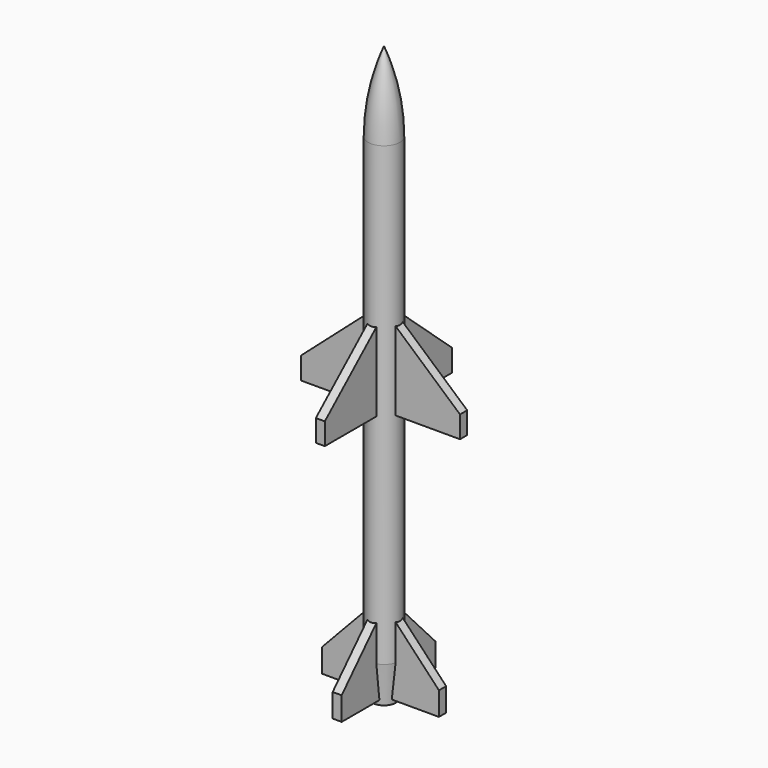
from build123d import *

# Parameters (mm, degrees)
F4_DEPTH     = 0.2
F5_COUNT     = 4
F7_DEPTH     = 17.9166666667
F8_T4_ANGLE  = 180
F8_S5_R      = 0.7048611111
F8_T6_DEPTH  = 2
F8_T10_DEPTH = 0.263819099
F8_S11_R     = 0.7048611111
F8_T12_DEPTH = 2
F8_T16_DEPTH = 0.263819099
F8_S17_R     = 0.7048611111
F8_T18_DEPTH = 2


# Not quite as in the source:
# - a fillet or chamfer that OpenCascade refuses, or shapes differently, is made with other operations: its cross-section is extruded or revolved along the edge and cut away or added
# - a feature names something its author has since deleted; it is built from what else it names


with BuildPart() as f2:
    # F1 (on Front) → F2 (revolve)
    with BuildSketch(Plane.XZ):
        with BuildLine():
            Line((0, 25.5555555556), (0, 0))
            Line((0, 0), (0.5208333333, 0))
            Line((0.5208333333, 0), (0.7048611111, 1.7013888889))
            Line((0.7048611111, 1.7013888889), (0.7048611111, 22.0138888889))
            ThreePointArc((0.7048611111, 22.0138888889), (0.5269346389, 23.8194519564), (0, 25.5555555556))
        make_face()
    revolve(axis=Axis((0, 0, 12.7777777778), (0, 0, 1)))

    # F3 (on Front) → F4 (join, symmetric)
    with BuildSketch(Plane.XZ):
        Polygon((0, 1.7013888889), (0, 0.2083333333), (2.6041666667, 0.2083333333), (2.6041666667, 1.25), (0.4, 3.5871419866), (0.4, 11.3888888889), (3.5416666667, 11.3888888889), (3.5416666667, 12.3611111111), (0, 15.4822861417), align=None)
    extrude(amount=F4_DEPTH, both=True)

    # F5: F2 ×4 about axis
    f5_axis = Axis((0, 0, 1.7013888889), (0, 0, 1))


with BuildPart() as f2_1:
    add(f2.part)
    for i in range(1, F5_COUNT):
        add(f2.part.rotate(f5_axis, i * 360 / F5_COUNT))

    # F6 (on face) → F7 (join)
    with BuildSketch(Plane(origin=(0, 0, 0), x_dir=(1, 0, 0), z_dir=(0, 0, -1))):
        with BuildLine():
            Line((-0.3928371007, -0.589255651), (-0.0580600084, -0.2544785587))
            Line((-0.0580600084, -0.2544785587), (-0.2544785587, -0.0580600084))
            Line((-0.2544785587, -0.0580600084), (-0.589255651, -0.3928371007))
            ThreePointArc((-0.589255651, -0.3928371007), (-0.589255651, -0.589255651), (-0.3928371007, -0.589255651))
        make_face()
    extrude(amount=-F7_DEPTH)

    # F8: fillet of radius 0.1041666667 on 1 edges, made by hand


with BuildPart() as f8_tool2:
    # F8_s3 → F8_t4 (revolve)
    with BuildSketch(Plane(origin=(-0.4910463758, 0.4910463758, 0), x_dir=(0, 0, 1), z_dir=(0.7071067812, -0.7071067812, 0))):
        with BuildLine():
            ThreePointArc((17.9166666667, 0.0347222222), (17.8861569564, 0.1083791786), (17.8125, 0.1388888889))
            Line((17.8125, 0.1388888889), (17.9166666667, 0.1388888889))
            Line((17.9166666667, 0.1388888889), (17.9166666667, 0.0347222222))
        make_face()
    revolve(axis=Axis((-0.4910463758, 0.4910463758, 17.9166666667), (0, 0, -1)), revolution_arc=F8_T4_ANGLE)

    # F8_s5 → F8_t6 (cut, symmetric)
    with BuildSketch(Plane.XY.offset(17.9)):
        Circle(F8_S5_R)
    extrude(amount=F8_T6_DEPTH, both=True, mode=Mode.SUBTRACT)


with BuildPart() as f2_2:
    add(f2_1.part)

    # F8_t1: cut F8_tool2
    add(f8_tool2.part, mode=Mode.SUBTRACT)


with BuildPart() as f8_tool8:
    # F8_s9 → F8_t10 (new body)
    with BuildSketch(Plane(origin=(-0.3044981019, 0.3044981019, 0), x_dir=(0, 0, 1), z_dir=(-0.7071067812, 0.7071067812, 0))):
        with BuildLine():
            ThreePointArc((17.9166666667, -0.0347222222), (17.8861569564, -0.1083791786), (17.8125, -0.1388888889))
            Line((17.8125, -0.1388888889), (17.9166666667, -0.1388888889))
            Line((17.9166666667, -0.1388888889), (17.9166666667, -0.0347222222))
        make_face()
    extrude(amount=F8_T10_DEPTH)

    # F8_s11 → F8_t12 (cut, symmetric)
    with BuildSketch(Plane.XY.offset(17.9)):
        Circle(F8_S11_R)
    extrude(amount=F8_T12_DEPTH, both=True, mode=Mode.SUBTRACT)


with BuildPart() as f2_3:
    add(f2_2.part)

    # F8_t7: cut F8_tool8
    add(f8_tool8.part, mode=Mode.SUBTRACT)


with BuildPart() as f8_tool14:
    # F8_s15 → F8_t16 (new body)
    with BuildSketch(Plane(origin=(-0.4910463758, 0.4910463758, 0), x_dir=(0, 0, 1), z_dir=(0.7071067812, -0.7071067812, 0))):
        with BuildLine():
            ThreePointArc((17.8125, -0.1388888889), (17.8861569564, -0.1083791786), (17.9166666667, -0.0347222222))
            Line((17.9166666667, -0.0347222222), (17.9166666667, -0.1388888889))
            Line((17.9166666667, -0.1388888889), (17.8125, -0.1388888889))
        make_face()
    extrude(amount=F8_T16_DEPTH)

    # F8_s17 → F8_t18 (cut, symmetric)
    with BuildSketch(Plane.XY.offset(17.9)):
        Circle(F8_S17_R)
    extrude(amount=F8_T18_DEPTH, both=True, mode=Mode.SUBTRACT)


with BuildPart() as f2_4:
    add(f2_3.part)

    # F8_t13: cut F8_tool14
    add(f8_tool14.part, mode=Mode.SUBTRACT)


solid = f2_4.part
